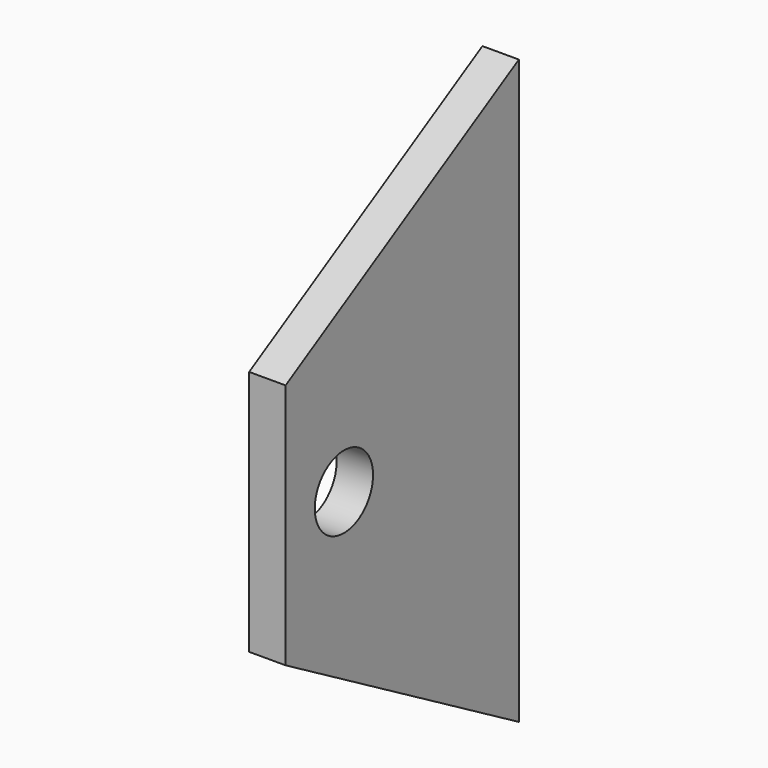
from build123d import *

# Parameters (mm, degrees)
F1_DEPTH = 6.35
F2_D     = 12.7


# Not quite as in the source:
# - a feature names something its author has since deleted; it is built from what else it names


with BuildPart() as f1:
    # F0 (on Right) → F1 (new body)
    with BuildSketch(Plane.YZ):
        Polygon((-73.2459126534, -2.6395988316), (-73.2459126534, -45.580811482), (-22.4459126534, -74.9102051568), (-22.4459126534, 26.6897948432), align=None)
    extrude(amount=F1_DEPTH)

    # F2 (through all)
    with Locations(Plane(origin=(0, 0, 0), x_dir=(0, 1, 0), z_dir=(-1, 0, 0))):
        with Locations((-60.5459126534, 24.1152988316)):
            Hole(F2_D / 2)


solid = f1.part
